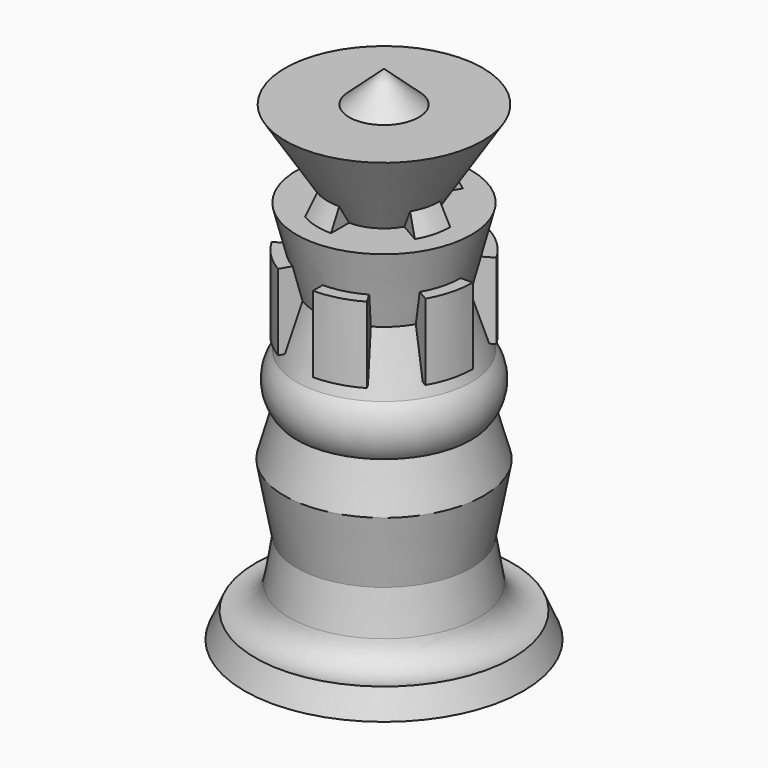
from build123d import *

# Parameters (mm, degrees)
F2_W            = 4.3805325404
F2_H            = 13.738937676
F3_ANGLE        = 30
F3_COPIES_COUNT = 6
F5_ANGLE        = 30
F5_COPIES_COUNT = 4


# Not quite as in the source:
# - a pattern or mirror of a feature is missing from the dataset's text; its kind, count and spacing are read off the source's solid


with BuildPart() as f1:
    # F0 (on Front) → F1 (revolve)
    with BuildSketch(Plane.XZ):
        Polygon((0, 72.776556015), (0, 67.1017691493), (6.2909605913, 67.1017691493), align=None)
        Polygon((0, 67.1017691493), (0, 51.4894537628), (7.8760384344, 51.4894537628), (17.8207978606, 67.1017691493), (6.2909605913, 67.1017691493), align=None)
        with BuildLine():
            Line((0, 51.4894537628), (0, -17.9203543812))
            Line((0, -17.9203543812), (25.1880511642, -17.9203543812))
            Line((25.1880511642, -17.9203543812), (23.1969021261, -13.3407087997))
            ThreePointArc((23.1969021261, -13.3407087997), (19.2033042996, -12.428933787), (17.024340108, -8.9601771906))
            Line((17.024340108, -8.9601771906), (15.7520768689, -1.4651455679))
            Line((15.7520768689, -1.4651455679), (18.0199127644, 10.7748573646))
            Line((18.0199127644, 10.7748573646), (15.7520768689, 18.9159307629))
            ThreePointArc((15.7520768689, 18.9159307629), (17.3860110627, 23.4955772758), (15.7520768689, 28.0752237886))
            Line((15.7520768689, 28.0752237886), (12.3262992129, 38.1487458944))
            Line((12.3262992129, 38.1487458944), (15.7520768689, 51.4894537628))
            Line((15.7520768689, 51.4894537628), (7.8760384344, 51.4894537628))
            Line((7.8760384344, 51.4894537628), (0, 51.4894537628))
        make_face()
    revolve(axis=Axis((0, 0, 27.4281008169), (0, 0, -1)))

    # F2 (on Front) → F3 (revolve)
    with BuildSketch(Plane.XZ):
        with Locations((13.8384955935, 37.1349565685)):
            Rectangle(F2_W, F2_H)
    f3 = revolve(axis=Axis((0, 0, 27.4281008169), (0, 0, -1)), revolution_arc=F3_ANGLE)

    # F3_copies: F3 ×6 about axis
    f3_copies_axis = Axis((0, 0, 0), (0, 0, 1))
    for i in range(1, F3_COPIES_COUNT):
        add(f3.rotate(f3_copies_axis, i * 360 / F3_COPIES_COUNT))

    # F4 (on Front) → F5 (revolve)
    with BuildSketch(Plane.XZ):
        Polygon((12.8429187462, 49.7787632048), (8.263274096, 58.5398264229), (6.6703548655, 49.7787632048), align=None)
    f5 = revolve(axis=Axis((0, 0, 27.4281008169), (0, 0, -1)), revolution_arc=F5_ANGLE)

    # F5_copies: F5 ×4 about axis
    f5_copies_axis = Axis((0, 0, 0), (0, 0, 1))
    for i in range(1, F5_COPIES_COUNT):
        add(f5.rotate(f5_copies_axis, i * 360 / F5_COPIES_COUNT))


solid = f1.part
